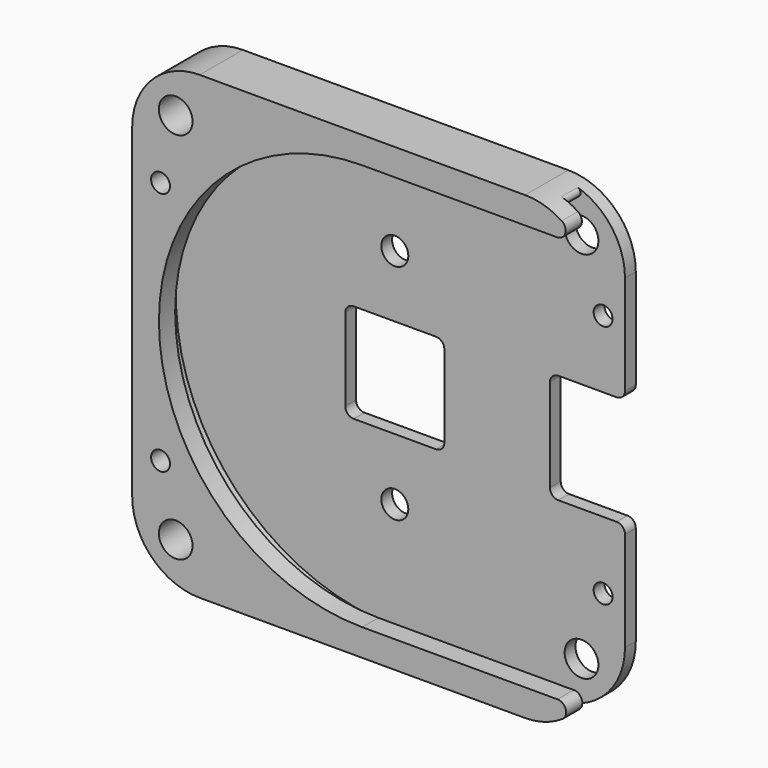
from build123d import *

# Parameters (mm, degrees)
F0_W         = 43.307
F0_H         = 43.307
F1_DEPTH     = 1.27
F3_DEPTH     = 3.175
F5_DEPTH     = 1.905
F6_R         = 0.889
F7_DEPTH     = 5.081
F8_W         = 9.3218
F8_H         = 9.3218
F8_W_2       = 7.0612
F8_H_2       = 10.3124
F10_DEPTH    = 1.27
F11_D        = 3.175
F14_D        = 2.54
F15_R        = 6.35
F16_T4_DEPTH = 12.7851645967
F16_T9_DEPTH = 12.8907938144
F17_R        = 0.7874
F18_D        = 3.175
F18_DEPTH    = 3.175
F18_TIP      = 0.9538662327
F19_T4_DEPTH = 6.3848359064
F19_T9_DEPTH = 6.2809008493


# Not quite as in the source:
# - a fillet or chamfer that OpenCascade refuses, or shapes differently, is made with other operations: its cross-section is extruded or revolved along the edge and cut away or added


with BuildPart() as f1:
    # F0 (on Front) → F1 (new body)
    with BuildSketch(Plane.XZ):
        with Locations((21.6535, 21.6535)):
            Rectangle(F0_W, F0_H)
    extrude(amount=F1_DEPTH)

    # F2 (on Front) → F3 (join)
    with BuildSketch(Plane.XZ):
        with BuildLine():
            Line((43.307, 43.307), (0, 43.307))
            Line((0, 43.307), (0, 0))
            Line((0, 0), (43.307, 0))
            Line((43.307, 0), (43.307, 1.0922))
            Line((43.307, 1.0922), (21.6408, 1.0922))
            ThreePointArc((21.6408, 1.0922), (1.0668, 21.6662), (21.6408, 42.2402))
            Line((21.6408, 42.2402), (43.307, 42.2402))
            Line((43.307, 42.2402), (43.307, 43.307))
        make_face()
    extrude(amount=F3_DEPTH)

    # F4 (on face) → F5 (join)
    with BuildSketch(Plane.XZ.offset(3.175)):
        with BuildLine():
            Line((43.307, 43.307), (0, 43.307))
            Line((0, 43.307), (0, 0))
            Line((0, 0), (43.307, 0))
            Line((43.307, 0), (43.307, 2.54))
            Line((43.307, 2.54), (21.6408, 2.54))
            ThreePointArc((21.6408, 2.54), (2.5146, 21.6662), (21.6408, 40.7924))
            Line((21.6408, 40.7924), (43.307, 40.7924))
            Line((43.307, 40.7924), (43.307, 43.307))
        make_face()
    extrude(amount=F5_DEPTH)

    # F6 (on face) → F7 (cut, through all)
    with BuildSketch(Plane(origin=(0, 0, 0), x_dir=(-1, 0, 0), z_dir=(0, 1, 0))):
        with Locations((-41.2496, 33.1724)):
            Circle(F6_R)
        with Locations((-2.667, 33.1724)):
            Circle(F6_R)
        with Locations((-41.2496, 10.16)):
            Circle(F6_R)
        with Locations((-2.667, 10.16)):
            Circle(F6_R)
    extrude(amount=-F7_DEPTH, mode=Mode.SUBTRACT)

    # F8 (on face) → F10 (cut, through all)
    with BuildSketch(Plane.XZ.offset(1.27)):
        with Locations((21.6535, 21.6535)):
            Rectangle(F8_W, F8_H)
        with Locations((39.7764, 21.6662)):
            Rectangle(F8_W_2, F8_H_2)
    extrude(amount=-F10_DEPTH, mode=Mode.SUBTRACT)

    # F11 (through all)
    with Locations(Plane(origin=(0, 0, 0), x_dir=(-1, 0, 0), z_dir=(0, 1, 0))):
        with Locations((-4.0894, 39.2176), (-4.0894, 4.0894)):
            Hole(F11_D / 2)

    # F14 (through all)
    with Locations(Plane(origin=(0, 0, 0), x_dir=(-1, 0, 0), z_dir=(0, 1, 0))):
        with Locations((-21.6535, 32.1564), (-21.6535, 11.176)):
            Hole(F14_D / 2)

    # F15
    f15_edges = [f1.edges().sort_by_distance(p)[0] for p in [
        (0, -2.54, 43.307),
        (43.307, -2.54, 43.307),
        (43.307, -2.54, 0),
        (0, -2.54, 0),
    ]]
    fillet(f15_edges, radius=F15_R)

    # F16: fillet of radius 0.8128 on 2 edges, made by hand


with BuildPart() as f16_tool2:
    # F16_s3 → F16_t4 (new body)
    with BuildSketch(Plane.XZ.offset(10.5200822984)):
        with BuildLine():
            ThreePointArc((40.005, 2.54), (40.7835212046, 1.9607563614), (40.452412844, 1.0486238532))
            ThreePointArc((40.452412844, 1.0486238532), (41.3090658387, 1.7259300464), (42.037, 2.54))
            Line((42.037, 2.54), (40.005, 2.54))
        make_face()
    extrude(amount=-F16_T4_DEPTH)

    split(bisect_by=Plane.XZ.offset(1.27), keep=Keep.TOP)


with BuildPart() as f1_1:
    add(f1.part)

    # F16_t1: cut F16_tool2
    add(f16_tool2.part, mode=Mode.SUBTRACT)


with BuildPart() as f16_tool7:
    # F16_s8 → F16_t9 (new body)
    with BuildSketch(Plane.XZ.offset(10.5728969072)):
        with BuildLine():
            ThreePointArc((39.9661228955, 40.7924), (40.7456166441, 41.374910322), (40.4078290086, 42.2875045872))
            ThreePointArc((40.4078290086, 42.2875045872), (41.2779959557, 41.6101165847), (42.0178504068, 40.7924))
            Line((42.0178504068, 40.7924), (39.9661228955, 40.7924))
        make_face()
    extrude(amount=-F16_T9_DEPTH)

    split(bisect_by=Plane.XZ.offset(1.27), keep=Keep.TOP)


with BuildPart() as f1_2:
    add(f1_1.part)

    # F16_t6: cut F16_tool7
    add(f16_tool7.part, mode=Mode.SUBTRACT)

    # F17
    f17_edges = [f1_2.edges().sort_by_distance(p)[0] for p in [
        (43.307, -0.635, 26.8224),
        (36.2458, -0.635, 26.8224),
        (16.9926, -0.635, 26.3144),
        (16.9926, -0.635, 16.9926),
        (26.3144, -0.635, 16.9926),
        (43.307, -0.635, 16.51),
        (36.2458, -0.635, 16.51),
        (26.3144, -0.635, 26.3144),
    ]]
    fillet(f17_edges, radius=F17_R)

    # F18
    with Locations(Plane(origin=(0, 0, 0), x_dir=(-1, 0, 0), z_dir=(0, 1, 0))):
        with Locations((-39.2176, 4.0894), (-39.2176, 39.2176)):
            Hole(F18_D / 2, depth=F18_DEPTH)
            with Locations((0, 0, -(F18_DEPTH + F18_TIP / 2))):  # 118° drill point
                Cone(0, F18_D / 2, F18_TIP, mode=Mode.SUBTRACT)

    # F19: fillet of radius 0.396875 on 2 edges, made by hand


with BuildPart() as f19_tool2:
    # F19_s3 → F19_t4 (new body)
    with BuildSketch(Plane.XZ.offset(-3.2098359064)):
        with BuildLine():
            ThreePointArc((38.8580757032, 43.0157466667), (39.1315562434, 42.57697322), (38.7392584717, 42.2402))
            Line((38.7392584717, 42.2402), (38.7392584717, 42.2005125))
            Line((38.7392584717, 42.2005125), (40.4734874982, 42.2005125))
            Line((40.4734874982, 42.2005125), (40.4982611604, 42.2712058594))
            ThreePointArc((40.4982611604, 42.2712058594), (40.4293966899, 42.3208202408), (38.8699574263, 43.0536138333))
            Line((38.8699574263, 43.0536138333), (38.8580757032, 43.0157466667))
        make_face()
    extrude(amount=F19_T4_DEPTH)

    split(bisect_by=Plane.XZ.offset(1.27), keep=Keep.TOP)


with BuildPart() as f1_3:
    add(f1_2.part)

    # F19_t1: cut F19_tool2
    add(f19_tool2.part, mode=Mode.SUBTRACT)


with BuildPart() as f19_tool7:
    # F19_s8 → F19_t9 (new body)
    with BuildSketch(Plane.XZ.offset(-3.1059008493)):
        with BuildLine():
            ThreePointArc((38.9423609411, 0.3183466667), (39.2101451473, 0.7581600602), (38.8182758823, 1.0922))
            Line((38.8182758823, 1.0922), (38.8182758823, 1.1318875))
            Line((38.8182758823, 1.1318875), (40.5123646026, 1.1318875))
            Line((40.5123646026, 1.1318875), (40.5371382648, 1.0611941406))
            ThreePointArc((40.5371382648, 1.0611941406), (40.4742591743, 1.0154902523), (38.954769447, 0.2806488333))
            Line((38.954769447, 0.2806488333), (38.9423609411, 0.3183466667))
        make_face()
    extrude(amount=F19_T9_DEPTH)

    split(bisect_by=Plane.XZ.offset(1.27), keep=Keep.TOP)


with BuildPart() as f1_4:
    add(f1_3.part)

    # F19_t6: cut F19_tool7
    add(f19_tool7.part, mode=Mode.SUBTRACT)


solid = f1_4.part
